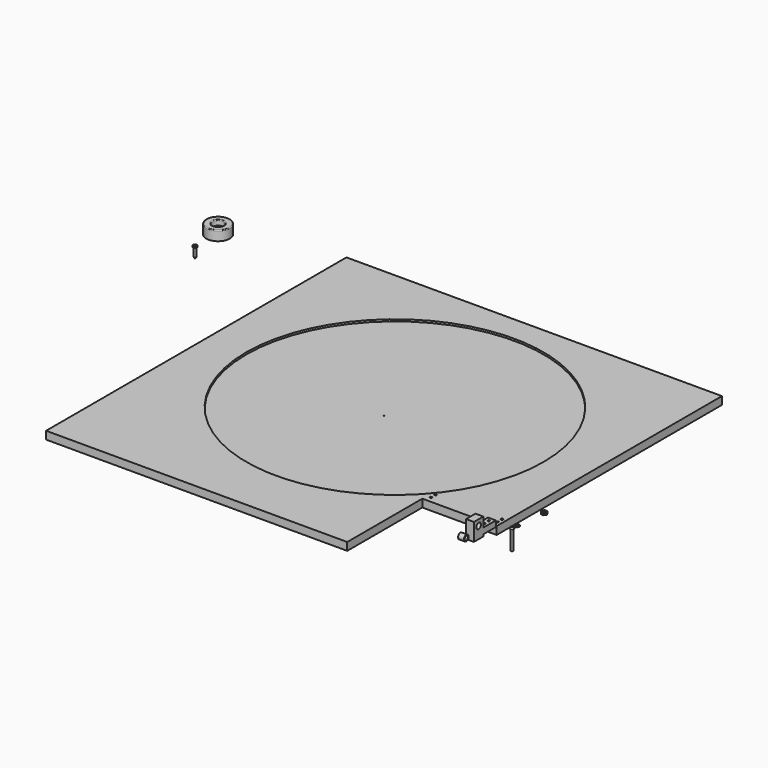
from build123d import *

# Parameters (mm, degrees)
F0_W      = 609.6
F0_H      = 609.6
F1_DEPTH  = 12.7
F2_R      = 19.05
F2_R_2    = 3.96875
F3_DEPTH  = 15.875
F4_R      = 9.525
F5_DEPTH  = 8.73125
F6_R      = 1.27
F7_R      = 8.8829111055
F7_R_2    = 4.8314193562
F8_DEPTH  = 0.79375
F9_R      = 0.79375
F10_DEPTH = 9.525
F11_R     = 3.429
F12_DEPTH = 2.4638
F13_W     = 1.6747713089
F13_H     = 0.8103847504
F13_W_2   = 1.0265111923
F13_H_2   = 2.1070092916
F13_W_3   = 1.8638670444
F13_H_3   = 2.0799934864
F14_DEPTH = 1.778
F16_R     = 1.7526
F17_DEPTH = 14.2875
F18_R     = 1.7148049935
F19_DEPTH = 1.5875
F19_TAPER = 30
F20_R     = 241.3
F21_DEPTH = 3.175
F22_W     = 120.65
F22_H     = 152.4
F23_DEPTH = 25.4
F24_R     = 1.7859375
F25_DEPTH = 25.4
F26_W     = 12.7
F26_H     = 44.45
F26_R     = 1.7859375
F27_DEPTH = 12.7
F28_W     = 12.7
F28_H     = 19.05
F29_DEPTH = 15.875
F30_R     = 4.7625
F31_DEPTH = 25.4
F32_R     = 4.7625
F32_R_2   = 3.175
F33_DEPTH = 9.525
F34_R     = 3.302
F35_DEPTH = 2.6162
F36_W     = 1.8160045147
F36_H     = 0.8614510298
F36_W_2   = 0.9312927723
F36_H_2   = 1.9789785147
F36_W_3   = 1.6297399998
F36_H_3   = 1.9324123859
F37_DEPTH = 2.286
F39_R     = 1.7526
F40_DEPTH = 31.75
F41_R     = 3.9624
F41_R_2   = 1.9812
F42_DEPTH = 0.635
F43_R     = 1.9812
F44_DEPTH = 2.778125
F45_R     = 3.175
F46_DEPTH = 4.7625
F47_W     = 12.7
F47_H     = 25.4
F48_DEPTH = 3.175


# Not quite as in the source:
# - a fillet or chamfer that OpenCascade refuses, or shapes differently, is made with other operations: its cross-section is extruded or revolved along the edge and cut away or added


with BuildPart() as f1:
    # F0 (on Top) → F1 (new body)
    with BuildSketch(Plane.XY):
        Rectangle(F0_W, F0_H)
    extrude(amount=-F1_DEPTH)

    # F9 (on face) → F10 (cut)
    with BuildSketch(Plane(origin=(0, 0, -12.7), x_dir=(1, 0, 0), z_dir=(0, 0, -1))):
        with Locations((-282.575, 282.575)):
            Circle(F9_R)
        with Locations((-282.575, -282.575)):
            Circle(F9_R)
        with Locations((282.575, -282.575)):
            Circle(F9_R)
        Circle(F9_R)
        with Locations((158.75, 282.575)):
            Circle(F9_R)
        with Locations((244.475, 282.575)):
            Circle(F9_R)
    extrude(amount=-F10_DEPTH, mode=Mode.SUBTRACT)

    # F20 (on face) → F21 (cut)
    with BuildSketch(Plane.XY):
        with Locations((0, 22.225)):
            Circle(F20_R)
    extrude(amount=-F21_DEPTH, mode=Mode.SUBTRACT)

    # F22 (on face) → F23 (cut)
    with BuildSketch(Plane.XY):
        with Locations((244.475, -228.6)):
            Rectangle(F22_W, F22_H)
    extrude(amount=-F23_DEPTH, mode=Mode.SUBTRACT)

    # F24 (on face) → F25 (cut)
    with BuildSketch(Plane.XY):
        with Locations((190.5, -133.35)):
            Circle(F24_R)
        with Locations((190.5, -142.875)):
            Circle(F24_R)
        with Locations((298.45, -133.35)):
            Circle(F24_R)
        with Locations((298.45, -142.875)):
            Circle(F24_R)
    extrude(amount=-F25_DEPTH, mode=Mode.SUBTRACT)


with BuildPart() as f3:
    # F2 (on face) → F3 (new body)
    with BuildSketch(Plane.XY):
        with Locations((-471.3675379753, 252.475976944)):
            Circle(F2_R)
        with Locations((-471.3675379753, 252.475976944)):
            Circle(F2_R_2, mode=Mode.SUBTRACT)
    extrude(amount=F3_DEPTH)

    # F4 (on face) → F5 (cut)
    with BuildSketch(Plane.XY.offset(15.875)):
        with Locations((-471.3675379753, 252.475976944)):
            Circle(F4_R)
    extrude(amount=-F5_DEPTH, mode=Mode.SUBTRACT)

    # F6
    f6_edges = [f3.edges().sort_by_distance(p)[0] for p in [
        (-490.417538, 252.475977, 15.875),
        (-480.892538, 252.475977, 15.875),
    ]]
    fillet(f6_edges, radius=F6_R)

    # F7 (on face) → F8 (join)
    with BuildSketch(Plane.XY.offset(7.14375)):
        with Locations((-471.3675379753, 252.475976944)):
            Circle(F7_R)
        with Locations((-471.3675379753, 252.475976944)):
            Circle(F7_R_2, mode=Mode.SUBTRACT)
    extrude(amount=F8_DEPTH)


with BuildPart() as f12:
    # F11 (on face) → F12 (new body)
    with BuildSketch(Plane.XY):
        with Locations((-472.5285470486, 207.1487307549)):
            Circle(F11_R)
    extrude(amount=F12_DEPTH)

    # F13 (on face) → F14 (cut)
    with BuildSketch(Plane.XY.offset(2.4638)):
        with Locations((-473.9061892033, 207.0676982403)):
            Rectangle(F13_W, F13_H)
        with Locations((-472.5555479527, 208.5263952613)):
            Rectangle(F13_W_2, F13_H_2)
        with Locations((-472.5555479527, 207.0676982403)):
            Rectangle(F13_W_2, F13_H)
        with Locations((-471.1103588343, 207.0676982403)):
            Rectangle(F13_W_3, F13_H)
        with Locations((-472.5555479527, 205.6225091219)):
            Rectangle(F13_W_2, F13_H_3)
    extrude(amount=-F14_DEPTH, mode=Mode.SUBTRACT)

    # F15: fillet of radius 1.016 on 1 edges, made by hand

    # F15_s1 → F15_t2 (revolve, cut)
    with BuildSketch(Plane.XZ.offset(-207.1487307549)):
        with BuildLine():
            ThreePointArc((-469.0995470486, 1.4478), (-469.3971265589, 2.1662204897), (-470.1155470486, 2.4638))
            Line((-470.1155470486, 2.4638), (-469.0995470486, 2.4638))
            Line((-469.0995470486, 2.4638), (-469.0995470486, 1.4478))
        make_face()
    revolve(axis=Axis((-472.5285470486, 207.1487307549, 2.4638), (0, 0, 1)), mode=Mode.SUBTRACT)

    # F16 (on face) → F17 (join)
    with BuildSketch(Plane(origin=(0, 0, 0), x_dir=(1, 0, 0), z_dir=(0, 0, -1))):
        with Locations((-472.5285470486, -207.1487307549)):
            Circle(F16_R)
    extrude(amount=F17_DEPTH)

    # F18 (on face) → F19 (join)
    with BuildSketch(Plane(origin=(0, 0, -14.2875), x_dir=(1, 0, 0), z_dir=(0, 0, -1))):
        with Locations((-472.5285470486, -207.1487307549)):
            Circle(F18_R)
    extrude(amount=F19_DEPTH, taper=F19_TAPER)


with BuildPart() as f27:
    # F26 (on face) → F27 (new body)
    with BuildSketch(Plane.XY.offset(-3.175)):
        with Locations((299.2969304323, -177.3378157832)):
            Rectangle(F26_W, F26_H)
        with Locations((299.2969304323, -170.9878157832)):
            Circle(F26_R, mode=Mode.SUBTRACT)
        with Locations((299.2969304323, -161.4628157832)):
            Circle(F26_R, mode=Mode.SUBTRACT)
    extrude(amount=F27_DEPTH)

    # F28 (on face) → F29 (join)
    with BuildSketch(Plane.XY.offset(9.525)):
        with Locations((299.2969304323, -190.0378157832)):
            Rectangle(F28_W, F28_H)
    extrude(amount=F29_DEPTH)

    # F30 (on face) → F31 (cut)
    with BuildSketch(Plane.YZ.offset(305.6469304323)):
        with Locations((-190.0378157832, 15.875)):
            Circle(F30_R)
    extrude(amount=-F31_DEPTH, mode=Mode.SUBTRACT)

    # F45 (on face) → F46 (cut)
    with BuildSketch(Plane(origin=(0, 0, -3.175), x_dir=(1, 0, 0), z_dir=(0, 0, -1))):
        with Locations((299.2969304323, 190.0378157832)):
            Circle(F45_R)
    extrude(amount=-F46_DEPTH, mode=Mode.SUBTRACT)

    # F47 (on face) → F48 (cut)
    with BuildSketch(Plane(origin=(0, 0, -3.175), x_dir=(1, 0, 0), z_dir=(0, 0, -1))):
        with Locations((299.2969304323, 167.8128157832)):
            Rectangle(F47_W, F47_H)
    extrude(amount=-F48_DEPTH, mode=Mode.SUBTRACT)


with BuildPart() as f33:
    # F32 (on face) → F33 (new body)
    with BuildSketch(Plane.YZ.offset(305.6469304323)):
        with Locations((-226.993098855, 16.5411494672)):
            Circle(F32_R)
        with Locations((-226.993098855, 16.5411494672)):
            Circle(F32_R_2, mode=Mode.SUBTRACT)
    extrude(amount=F33_DEPTH)


with BuildPart() as f35:
    # F34 (on face) → F35 (new body)
    with BuildSketch(Plane.XY):
        with Locations((324.1440951824, -145.285114646)):
            Circle(F34_R)
    extrude(amount=F35_DEPTH)

    # F36 (on face) → F37 (cut)
    with BuildSketch(Plane.XY.offset(2.6162)):
        with Locations((322.7704316378, -145.2501937747)):
            Rectangle(F36_W, F36_H)
        with Locations((324.1440802813, -143.8299790025)):
            Rectangle(F36_W_2, F36_H_2)
        with Locations((324.1440802813, -145.2501937747)):
            Rectangle(F36_W_2, F36_H)
        with Locations((325.4245966673, -145.2501937747)):
            Rectangle(F36_W_3, F36_H)
        with Locations((324.1440802813, -146.6471254826)):
            Rectangle(F36_W_2, F36_H_3)
    extrude(amount=-F37_DEPTH, mode=Mode.SUBTRACT)

    # F38: fillet of radius 2.54 on 1 edges, made by hand

    # F38_s1 → F38_t2 (revolve, cut)
    with BuildSketch(Plane.XZ.offset(145.285114646)):
        with BuildLine():
            ThreePointArc((327.4460951824, 0.0762), (326.7021464066, 1.8722512242), (324.9060951824, 2.6162))
            Line((324.9060951824, 2.6162), (327.4460951824, 2.6162))
            Line((327.4460951824, 2.6162), (327.4460951824, 0.0762))
        make_face()
    revolve(axis=Axis((324.1440951824, -145.285114646, 2.6162), (0, 0, 1)), mode=Mode.SUBTRACT)

    # F39 (on face) → F40 (join)
    with BuildSketch(Plane(origin=(0, 0, 0), x_dir=(1, 0, 0), z_dir=(0, 0, -1))):
        with Locations((324.1440951824, 145.285114646)):
            Circle(F39_R)
    extrude(amount=F40_DEPTH)


with BuildPart() as f42:
    # F41 (on face) → F42 (new body)
    with BuildSketch(Plane.XY):
        with Locations((323.5958218575, -134.8513066769)):
            Circle(F41_R)
        with Locations((323.5958218575, -134.8513066769)):
            Circle(F41_R_2, mode=Mode.SUBTRACT)
    extrude(amount=-F42_DEPTH)


with BuildPart() as f44:
    # F43 (on face) → F44 (new body)
    with BuildSketch(Plane.XY):
        Polygon((332.8111508927, -91.9929276752), (335.1391998381, -88.0453606938), (332.8845310219, -84.0554276752), (328.3018132602, -84.0130616379), (325.9737643148, -87.9606286192), (328.228433131, -91.9505616379), align=None)
        with Locations((330.5564820765, -88.0029946565)):
            Circle(F43_R, mode=Mode.SUBTRACT)
    extrude(amount=F44_DEPTH)


solid = Compound([f1.part, f3.part, f12.part, f27.part, f33.part, f35.part, f42.part, f44.part])
